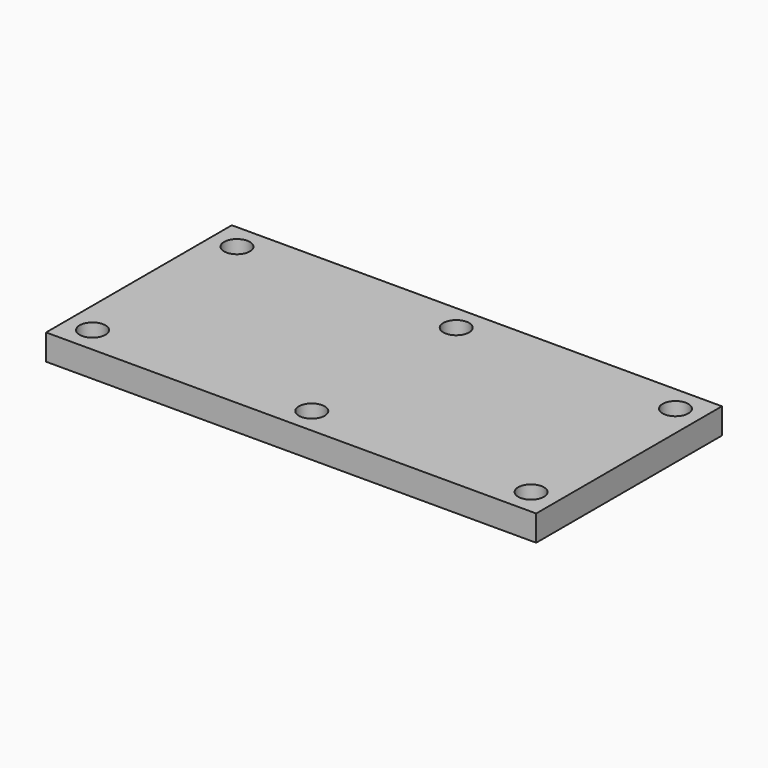
from build123d import *

# Parameters (mm, degrees)
F0_W     = 241.3
F0_H     = 114.3
F1_DEPTH = 12.7
F2_W     = 190.5
F2_H     = 63.5
F3_DEPTH = 12.7
F4_R     = 6.35
F5_DEPTH = 12.7


# Not quite as in the source:
# - a feature names something its author has since deleted; it is built from what else it names


with BuildPart() as f1:
    # F0 (on Top) → F1 (new body)
    with BuildSketch(Plane.XY):
        Rectangle(F0_W, F0_H)
    extrude(amount=F1_DEPTH)

    # F2 (on face) → F3 (join)
    with BuildSketch(Plane(origin=(0, 0, 0), x_dir=(1, 0, 0), z_dir=(0, 0, -1))):
        Rectangle(F2_W, F2_H)
    extrude(amount=F3_DEPTH)

    # F4 (on face) → F5 (cut)
    with BuildSketch(Plane.XY.offset(12.7)):
        with Locations((-107.95, 44.45)):
            Circle(F4_R)
        with Locations((-107.95, -44.45)):
            Circle(F4_R)
        with Locations((107.95, -44.45)):
            Circle(F4_R)
        with Locations((107.95, 44.45)):
            Circle(F4_R)
        with Locations((0, 44.45)):
            Circle(F4_R)
        with Locations((0, -44.45)):
            Circle(F4_R)
    extrude(amount=-F5_DEPTH, mode=Mode.SUBTRACT)


solid = f1.part
